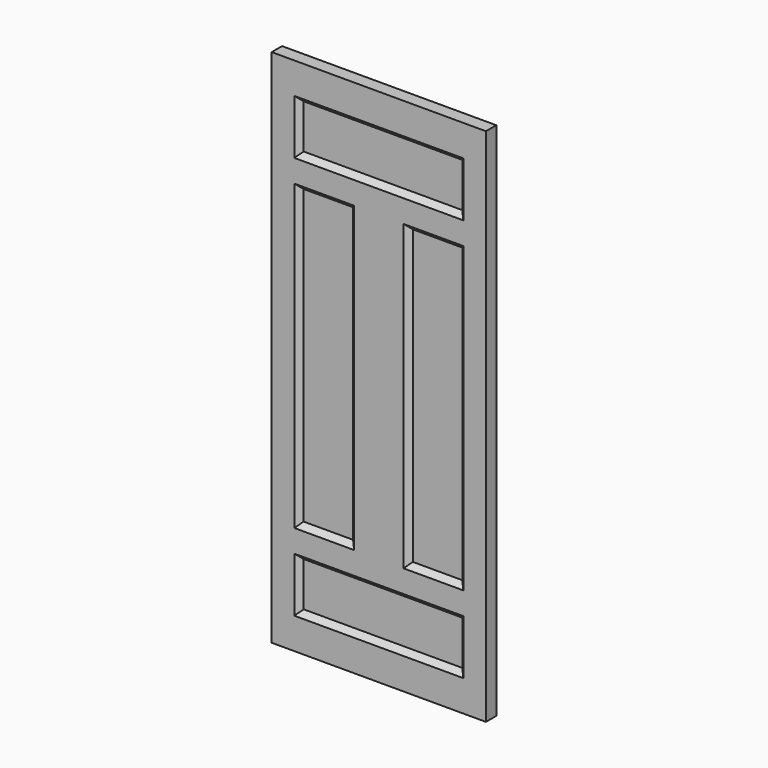
from build123d import *

# Parameters (mm, degrees)
F0_W     = 824
F0_H     = 2000
F1_DEPTH = 50
F2_W     = 650
F2_H     = 210
F2_W_2   = 230
F2_H_2   = 1166
F3_DEPTH = 20
F4_SIZE  = 19.99999


# Not quite as in the source:
# - a fillet or chamfer is up to 0.001 mm smaller than in the source, because OpenCascade refuses the exact size


with BuildPart() as f1:
    # F0 (on Front) → F1 (new body)
    with BuildSketch(Plane.XZ):
        Rectangle(F0_W, F0_H)
    extrude(amount=F1_DEPTH)

    # F2 (on face) → F3 (cut)
    with BuildSketch(Plane.XZ.offset(50)):
        with Locations((0, 775)):
            Rectangle(F2_W, F2_H)
        with Locations((-210, 0)):
            Rectangle(F2_W_2, F2_H_2)
        with Locations((210, 0)):
            Rectangle(F2_W_2, F2_H_2)
        with Locations((0, -775)):
            Rectangle(F2_W, F2_H)
    extrude(amount=-F3_DEPTH, mode=Mode.SUBTRACT)

    # F4 (size 20 in the source; OpenCascade refuses exactly that, so slightly less here)
    f4_edges = [f1.edges().sort_by_distance(p)[0] for p in [
        (-95, -30, 0),
        (-210, -30, 583),
        (-325, -30, 0),
        (-210, -30, -583),
        (210, -30, -583),
        (95, -30, 0),
        (325, -30, 0),
        (210, -30, 583),
        (0, -30, 880),
        (-325, -30, 775),
        (325, -30, 775),
        (0, -30, 670),
        (-325, -30, -775),
        (0, -30, -880),
        (325, -30, -775),
        (0, -30, -670),
    ]]
    chamfer(f4_edges, length=F4_SIZE)


solid = f1.part
